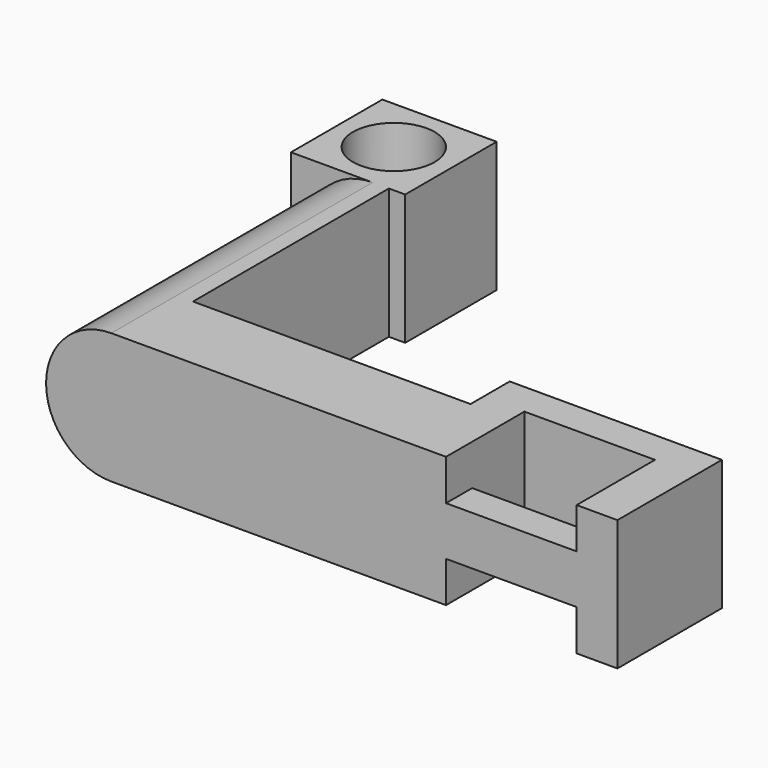
from build123d import *

# Parameters (mm, degrees)
F0_R     = 2.5
F0_W     = 8
F0_H     = 2
F1_DEPTH = 8
F2_W     = 8
F2_H     = 2.5
F3_DEPTH = 3
F4_R     = 3.99999


# Not quite as in the source:
# - a fillet or chamfer is up to 0.001 mm smaller than in the source, because OpenCascade refuses the exact size


with BuildPart() as f1:
    # F0 (on Top) → F1 (new body)
    with BuildSketch(Plane.XY):
        Polygon((-3.5, 10), (-2.5, 10), (2.5, 10), (3.5, 10), (3.5, 17), (-3.5, 17), align=None)
        with Locations((0, 13.5)):
            Circle(F0_R, mode=Mode.SUBTRACT)
        Polygon((-2.5, -10), (2.5, -10), (2.5, -5), (2.5, 10), (-2.5, 10), align=None)
        Polygon((2.5, -5), (2.5, -10), (22, -10), (22, -8), (22, -5), (19.5, -5), align=None)
        with Locations((26, -9)):
            Rectangle(F0_W, F0_H)
        Polygon((30, -8), (30, -10), (32.5, -10), (32.5, -5), (30, -5), align=None)
        Polygon((19.5, -4), (19.5, -5), (22, -5), (22, -4), (30, -4), (30, -5), (32.5, -5), (32.5, -2), (19.5, -2), align=None)
    extrude(amount=F1_DEPTH)

    # F2 (on face) → F3 (cut)
    with BuildSketch(Plane.XZ.offset(10)):
        with Locations((26, 6.75)):
            Rectangle(F2_W, F2_H)
        with Locations((26, 1.25)):
            Rectangle(F2_W, F2_H)
    extrude(amount=-F3_DEPTH, mode=Mode.SUBTRACT)

    # F4 (radius 4 in the source; OpenCascade refuses exactly that, so slightly less here)
    f4_edges = [f1.edges().sort_by_distance(p)[0] for p in [
        (-2.5, 0, 8),
        (-2.5, 0, 0),
    ]]
    fillet(f4_edges, radius=F4_R)


solid = f1.part
